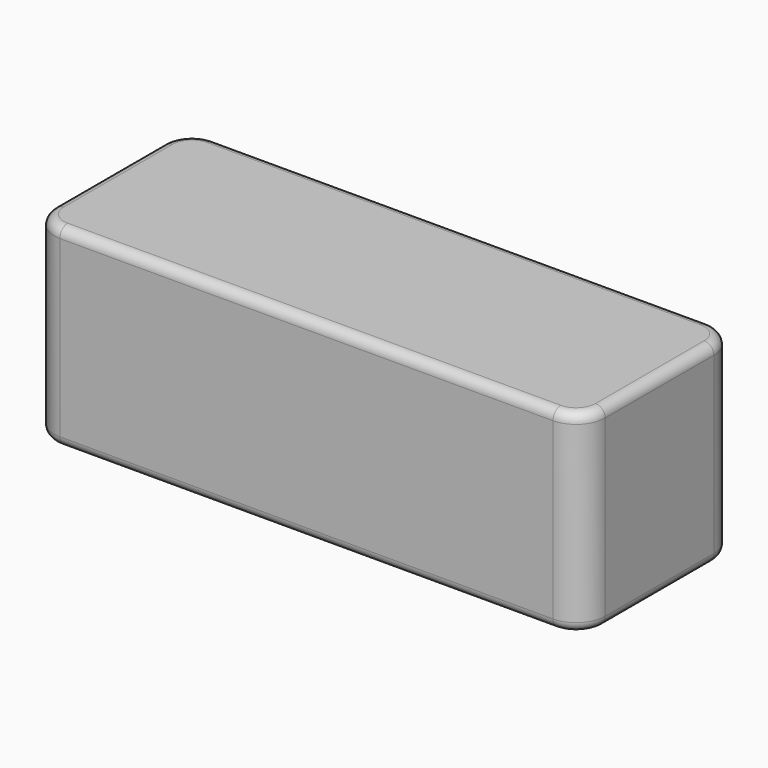
from build123d import *

# Parameters (mm, degrees)
F0_W         = 145
F0_H         = 51
F1_DEPTH     = 51
F2_R         = 2.54
F3_T1_DEPTH  = 51
F3_T4_ANGLE  = 90
F3_T6_ANGLE  = 90
F3_T8_ANGLE  = 90
F3_T10_ANGLE = 90
F3_T12_ANGLE = 90
F3_T14_ANGLE = 90
F3_T16_ANGLE = 90
F3_T18_ANGLE = 90


# Not quite as in the source:
# - a fillet or chamfer that OpenCascade refuses, or shapes differently, is made with other operations: its cross-section is extruded or revolved along the edge and cut away or added


with BuildPart() as f1:
    # F0 (on Top) → F1 (new body)
    with BuildSketch(Plane.XY):
        Rectangle(F0_W, F0_H)
    extrude(amount=F1_DEPTH)

    # F2
    f2_edges = [f1.edges().sort_by_distance(p)[0] for p in [
        (0, -25.5, 51),
        (0, 25.5, 51),
        (0, -25.5, 0),
        (0, 25.5, 0),
        (-72.5, 0, 0),
        (-72.5, 0, 51),
        (72.5, 0, 0),
        (72.5, 0, 51),
    ]]
    fillet(f2_edges, radius=F2_R)

    # F3: fillet of radius 7.62 on 4 edges, made by hand

    # F3_s2 → F3_t1 (cut)
    with BuildSketch(Plane.XY):
        with BuildLine():
            ThreePointArc((72.5, -17.88), (70.2681536726, -23.2681536726), (64.88, -25.5))
            Line((64.88, -25.5), (72.5, -25.5))
            Line((72.5, -25.5), (72.5, -17.88))
        make_face()
        with BuildLine():
            ThreePointArc((64.88, 25.5), (70.2681536726, 23.2681536726), (72.5, 17.88))
            Line((72.5, 17.88), (72.5, 25.5))
            Line((72.5, 25.5), (64.88, 25.5))
        make_face()
        with BuildLine():
            ThreePointArc((-72.5, -17.88), (-70.2681536726, -23.2681536726), (-64.88, -25.5))
            Line((-64.88, -25.5), (-72.5, -25.5))
            Line((-72.5, -25.5), (-72.5, -17.88))
        make_face()
        with BuildLine():
            ThreePointArc((-64.88, 25.5), (-70.2681536726, 23.2681536726), (-72.5, 17.88))
            Line((-72.5, 17.88), (-72.5, 25.5))
            Line((-72.5, 25.5), (-64.88, 25.5))
        make_face()
    extrude(amount=F3_T1_DEPTH, mode=Mode.SUBTRACT)

    # F3_s3 → F3_t4 (revolve, cut)
    with BuildSketch(Plane.XZ.offset(-17.88)):
        with BuildLine():
            ThreePointArc((-69.96, 0), (-71.7560512242, 0.7439487758), (-72.5, 2.54))
            Line((-72.5, 2.54), (-72.5, 0))
            Line((-72.5, 0), (-69.96, 0))
        make_face()
    revolve(axis=Axis((-64.88, 17.88, 0), (0, 0, -1)), revolution_arc=F3_T4_ANGLE, mode=Mode.SUBTRACT)

    # F3_s5 → F3_t6 (revolve, cut)
    with BuildSketch(Plane.YZ.offset(-64.88)):
        with BuildLine():
            ThreePointArc((22.96, 51), (24.7560512242, 50.2560512242), (25.5, 48.46))
            Line((25.5, 48.46), (25.5, 51))
            Line((25.5, 51), (22.96, 51))
        make_face()
    revolve(axis=Axis((-64.88, 17.88, 51), (0, 0, 1)), revolution_arc=F3_T6_ANGLE, mode=Mode.SUBTRACT)

    # F3_s7 → F3_t8 (revolve, cut)
    with BuildSketch(Plane.YZ.offset(-64.88)):
        with BuildLine():
            ThreePointArc((-22.96, 0), (-24.7560512242, 0.7439487758), (-25.5, 2.54))
            Line((-25.5, 2.54), (-25.5, 0))
            Line((-25.5, 0), (-22.96, 0))
        make_face()
    revolve(axis=Axis((-64.88, -17.88, 0), (0, 0, -1)), revolution_arc=F3_T8_ANGLE, mode=Mode.SUBTRACT)

    # F3_s9 → F3_t10 (revolve, cut)
    with BuildSketch(Plane.XZ.offset(17.88)):
        with BuildLine():
            ThreePointArc((-69.96, 51), (-71.7560512242, 50.2560512242), (-72.5, 48.46))
            Line((-72.5, 48.46), (-72.5, 51))
            Line((-72.5, 51), (-69.96, 51))
        make_face()
    revolve(axis=Axis((-64.88, -17.88, 51), (0, 0, 1)), revolution_arc=F3_T10_ANGLE, mode=Mode.SUBTRACT)

    # F3_s11 → F3_t12 (revolve, cut)
    with BuildSketch(Plane.YZ.offset(64.88)):
        with BuildLine():
            ThreePointArc((22.96, 0), (24.7560512242, 0.7439487758), (25.5, 2.54))
            Line((25.5, 2.54), (25.5, 0))
            Line((25.5, 0), (22.96, 0))
        make_face()
    revolve(axis=Axis((64.88, 17.88, 0), (0, 0, -1)), revolution_arc=F3_T12_ANGLE, mode=Mode.SUBTRACT)

    # F3_s13 → F3_t14 (revolve, cut)
    with BuildSketch(Plane.XZ.offset(-17.88)):
        with BuildLine():
            ThreePointArc((69.96, 51), (71.7560512242, 50.2560512242), (72.5, 48.46))
            Line((72.5, 48.46), (72.5, 51))
            Line((72.5, 51), (69.96, 51))
        make_face()
    revolve(axis=Axis((64.88, 17.88, 51), (0, 0, 1)), revolution_arc=F3_T14_ANGLE, mode=Mode.SUBTRACT)

    # F3_s15 → F3_t16 (revolve, cut)
    with BuildSketch(Plane.XZ.offset(17.88)):
        with BuildLine():
            ThreePointArc((69.96, 0), (71.7560512242, 0.7439487758), (72.5, 2.54))
            Line((72.5, 2.54), (72.5, 0))
            Line((72.5, 0), (69.96, 0))
        make_face()
    revolve(axis=Axis((64.88, -17.88, 0), (0, 0, -1)), revolution_arc=F3_T16_ANGLE, mode=Mode.SUBTRACT)

    # F3_s17 → F3_t18 (revolve, cut)
    with BuildSketch(Plane.YZ.offset(64.88)):
        with BuildLine():
            ThreePointArc((-22.96, 51), (-24.7560512242, 50.2560512242), (-25.5, 48.46))
            Line((-25.5, 48.46), (-25.5, 51))
            Line((-25.5, 51), (-22.96, 51))
        make_face()
    revolve(axis=Axis((64.88, -17.88, 51), (0, 0, 1)), revolution_arc=F3_T18_ANGLE, mode=Mode.SUBTRACT)


solid = f1.part
